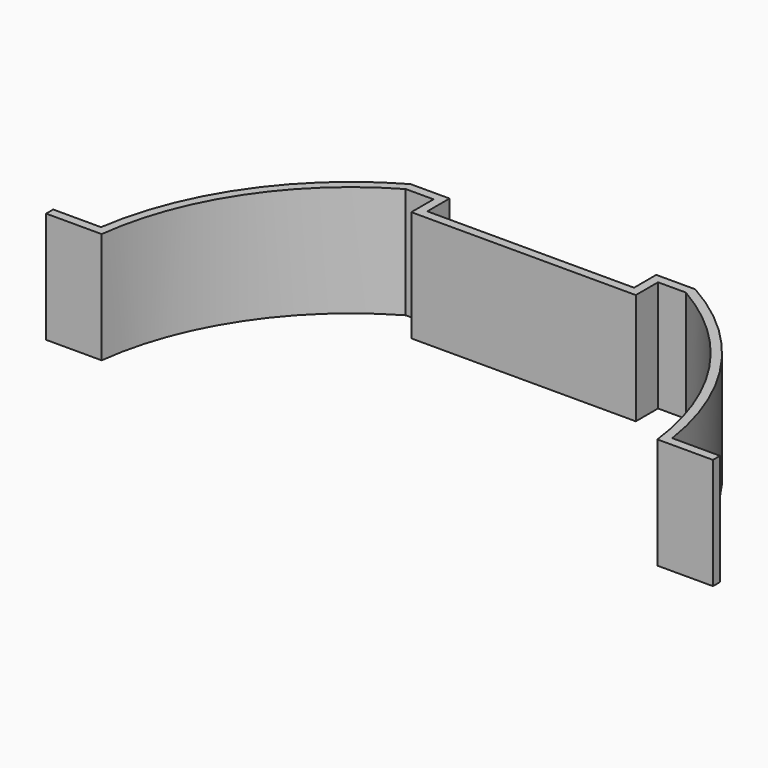
from build123d import *

# Parameters (mm, degrees)
F1_DEPTH = 25.4


# Not quite as in the source:
# - a pattern or mirror of a feature is missing from the dataset's text; its kind, count and spacing are read off the source's solid


with BuildPart() as f1:
    # F0 (on Top) → F1 (new body)
    with BuildSketch(Plane.XY):
        with BuildLine():
            Line((-25.654, 0), (0, 0))
            Line((0, 0), (0, 2.032))
            Line((0, 2.032), (-23.622, 2.032))
            Line((-23.622, 2.032), (-23.622, 8.382))
            Line((-23.622, 8.382), (-32.5398903871, 8.382))
            ThreePointArc((-32.5398903871, 8.382), (-54.4156625214, -11.5711123989), (-65.2763838561, -39.116))
            Line((-65.2763838561, -39.116), (-76.2, -39.116))
            Line((-76.2, -39.116), (-76.2, -41.148))
            Line((-76.2, -41.148), (-63.5, -41.148))
            ThreePointArc((-63.5, -41.148), (-53.3799799525, -13.6670774646), (-32.004, 6.35))
            Line((-32.004, 6.35), (-25.654, 6.35))
            Line((-25.654, 6.35), (-25.654, 0))
        make_face()
    extrude(amount=F1_DEPTH)

    # F1_copies: F1 across plane


with BuildPart() as f1_1:
    add(f1.part)
    add(f1.part.mirror(Plane(origin=(0, 0, 0), x_dir=(0, 0, 1), z_dir=(1, 0, 0))))


solid = f1_1.part
